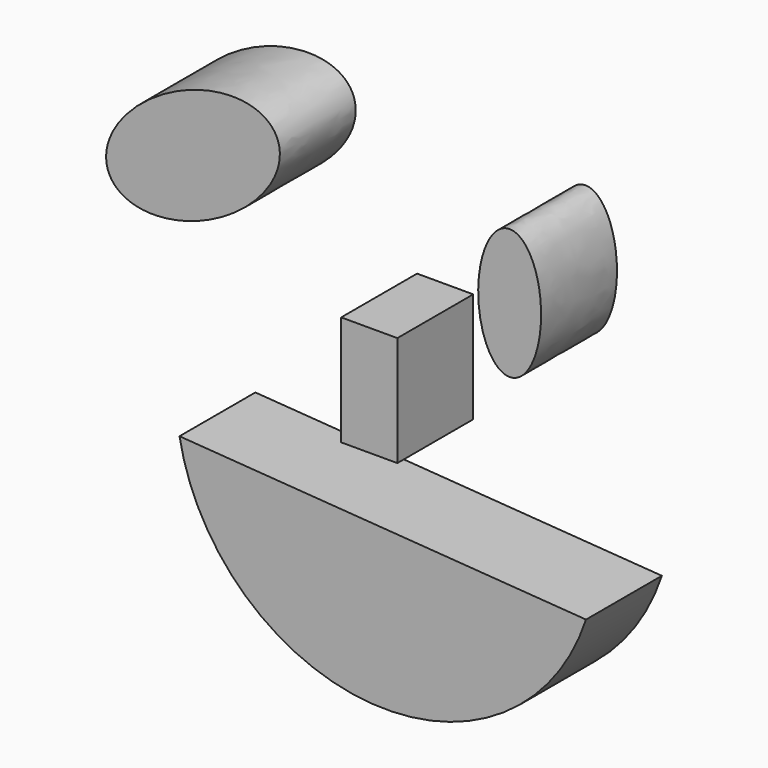
from build123d import *

# Parameters (mm, degrees)
F0_R     = 45.4286700741
F1_DEPTH = 12.7
F4_W     = 7.5197415426
F4_H     = 14.7386845201
F7_DEPTH = 25.4


# Not quite as in the source:
# - a feature of the source that left no trace in its solid (it failed there, or was rolled back) is left out


with BuildPart() as f1:
    # F0 (on Front) → F1 (new body)
    with BuildSketch(Plane.XZ):
        Circle(F0_R)
    extrude(amount=-F1_DEPTH)

    # F4 (on face) → F7 (intersect)
    with BuildSketch(Plane.XZ):
        with BuildLine():
            add(Edge.make_bspline(
                [(-12.4827632681, 26.0182898492), (-18.347071394, 36.8672613348), (-32.1087333857, 22.4190924464), (-45.8703953773, 7.9709235579), (-26.2444252597, 11.5701209607), (-6.6184551421, 15.1693183635), (-12.4827632681, 26.0182898492)],
                knots=[0, 0, 0, 2.0943951024, 2.0943951024, 4.1887902048, 4.1887902048, 6.2831853072, 6.2831853072, 6.2831853072], degree=2, weights=[1, 0.5, 1, 0.5, 1, 0.5, 1]))
        make_face()
        with BuildLine():
            add(Edge.make_bspline(
                [(18.7993403524, 7.670131512), (26.0974339214, 7.670131512), (22.4483871369, 20.7544737495), (18.7993403524, 33.8388159871), (15.1502935679, 20.7544737495), (11.5012467835, 7.670131512), (18.7993403524, 7.670131512)],
                knots=[0, 0, 0, 2.0943951024, 2.0943951024, 4.1887902048, 4.1887902048, 6.2831853072, 6.2831853072, 6.2831853072], degree=2, weights=[1, 0.5, 1, 0.5, 1, 0.5, 1]))
        make_face()
        Rectangle(F4_W, F4_H)
        with BuildLine():
            Line((29.0261879563, -17.5961833447), (-25.4167113453, -13.6859212071))
            ThreePointArc((-25.4167113453, -13.6859212071), (0.2825139058, -36.8351069939), (29.0261879563, -17.5961833447))
        make_face()
    extrude(amount=-F7_DEPTH, mode=Mode.INTERSECT)


solid = f1.part
